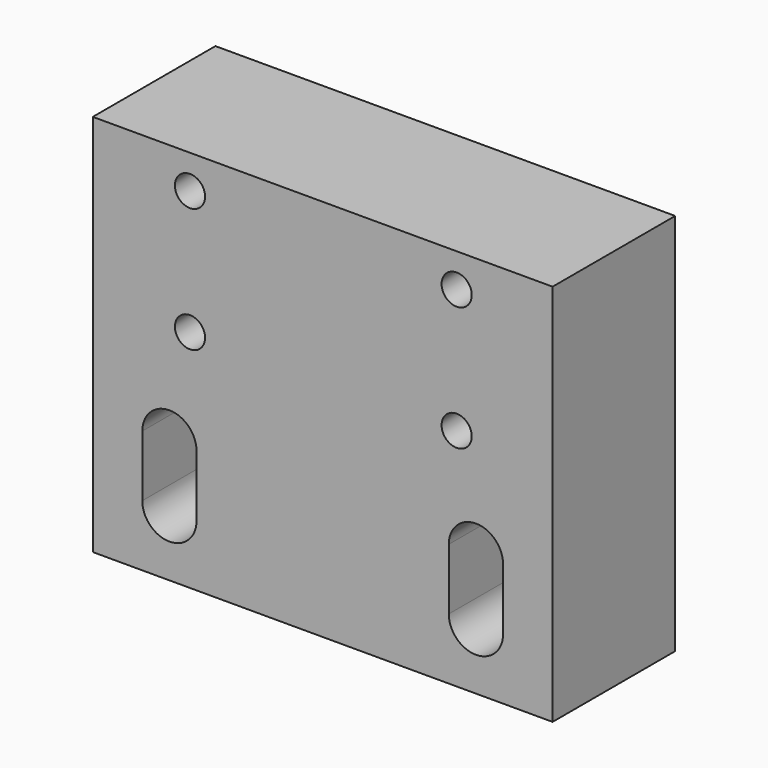
from build123d import *

# Parameters (mm, degrees)
F0_W     = 38.1
F0_H     = 31.75
F1_DEPTH = 6.35
F3_D     = 2.5
F5_DEPTH = 12.7


# Not quite as in the source:
# - a pattern or mirror of a feature is missing from the dataset's text; its kind, count and spacing are read off the source's solid


with BuildPart() as f1:
    # F0 (on Front) → F1 (new body, symmetric)
    with BuildSketch(Plane.XZ):
        Rectangle(F0_W, F0_H)
    extrude(amount=F1_DEPTH, both=True)

    # F3 (through all)
    with Locations(Plane.XZ.offset(6.35)):
        with Locations((-10.99693, 2.7813), (11.10107, 13.081), (-10.99693, 13.081), (11.10107, 2.7813)):
            Hole(F3_D / 2)

    # F4 (on face) → F5 (cut, through all)
    with BuildSketch(Plane.XZ.offset(6.35)):
        with BuildLine():
            ThreePointArc((-10.45, -5.715), (-12.7, -3.465), (-14.95, -5.715))
            Line((-14.95, -5.715), (-14.95, -10.795))
            ThreePointArc((-14.95, -10.795), (-12.7, -13.045), (-10.45, -10.795))
            Line((-10.45, -10.795), (-10.45, -5.715))
        make_face()
    f5 = extrude(amount=-F5_DEPTH, mode=Mode.SUBTRACT)

    # F5_copies: F5 across plane
    add(f5.mirror(Plane(origin=(0, 0, 0), x_dir=(0, 0, 1), z_dir=(1, 0, 0))), mode=Mode.SUBTRACT)


solid = f1.part
